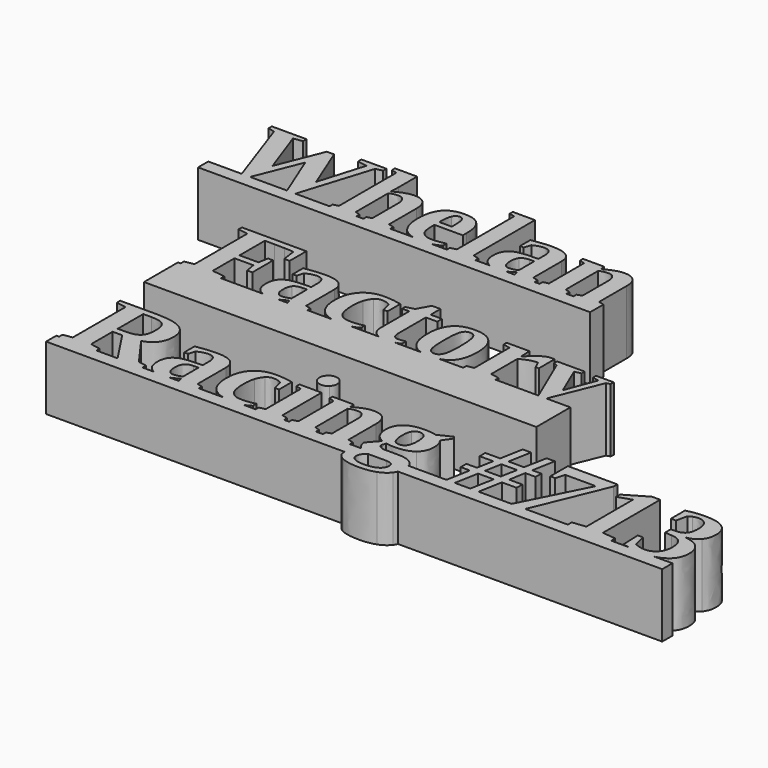
from build123d import *

# Parameters (mm, degrees)
F1_DEPTH = 15


with BuildPart() as f1:
    # F0 (on Top) → F1 (new body)
    with BuildSketch(Plane.XY):
        with BuildLine():
            Line((-29.6238354695, 35.7050479947), (-29.6238354695, 34.8109507725))
            Line((-29.6238354695, 34.8109507725), (-23.2913701918, 34.8109507725))
            Line((-23.2913701918, 34.8109507725), (-23.2913701918, 35.7050479947))
            Line((-23.2913701918, 35.7050479947), (-24.4545646362, 36.030568828))
            Line((-24.4545646362, 36.030568828), (-24.4545646362, 45.5661591058))
            add(Edge.make_bspline(
                [(-22.3929326918, 46.0262285502), (-23.4259188029, 46.0262285502), (-24.4545646362, 45.5661591058)],
                knots=[0, 0, 0, 1, 1, 1], degree=2))
            add(Edge.make_bspline(
                [(-21.0170646362, 45.3903778558), (-21.4988354695, 46.0262285502), (-22.3929326918, 46.0262285502)],
                knots=[0, 0, 0, 1, 1, 1], degree=2))
            add(Edge.make_bspline(
                [(-20.5352938029, 43.6130341058), (-20.5352938029, 44.7545271614), (-21.0170646362, 45.3903778558)],
                knots=[0, 0, 0, 1, 1, 1], degree=2))
            Line((-20.5352938029, 43.6130341058), (-20.5352938029, 36.030568828))
            Line((-20.5352938029, 36.030568828), (-21.6767868584, 35.7050479947))
            Line((-21.6767868584, 35.7050479947), (-21.6767868584, 34.8109507725))
            Line((-21.6767868584, 34.8109507725), (-15.3399813029, 34.8109507725))
            Line((-15.3399813029, 34.8109507725), (-15.3399813029, 35.7050479947))
            Line((-15.3399813029, 35.7050479947), (-16.6160229695, 36.030568828))
            Line((-16.6160229695, 36.030568828), (-16.6160229695, 44.1425479947))
            add(Edge.make_bspline(
                [(-20.1446688029, 47.9012285502), (-16.6160229695, 47.9012285502), (-16.6160229695, 44.1425479947)],
                knots=[0, 0, 0, 1, 1, 1], degree=2))
            add(Edge.make_bspline(
                [(-23.6038701918, 46.9246660502), (-21.6767868584, 47.9012285502), (-20.1446688029, 47.9012285502)],
                knots=[0, 0, 0, 1, 1, 1], degree=2))
            Line((-23.6038701918, 46.9246660502), (-24.537029914, 46.4472354947))
            add(Edge.make_bspline(
                [(-24.4545646362, 48.5652910502), (-24.4545646362, 47.671193828), (-24.537029914, 46.4472354947)],
                knots=[0, 0, 0, 1, 1, 1], degree=2))
            Line((-24.4545646362, 48.5652910502), (-24.4545646362, 54.0861243836))
            Line((-24.4545646362, 54.0861243836), (-29.6802590806, 54.0861243836))
            Line((-29.6802590806, 54.0861243836), (-29.6802590806, 53.1876868836))
            Line((-29.6802590806, 53.1876868836), (-28.3781757473, 52.8621660502))
            Line((-28.3781757473, 52.8621660502), (-28.3781757473, 36.030568828))
            Line((-28.3781757473, 36.030568828), (-29.6238354695, 35.7050479947))
        make_face()
        with BuildLine():
            Line((-23.2913701918, 34.8109507725), (-29.6238354695, 34.8109507725))
            Line((-29.6238354695, 34.8109507725), (-37.6563465286, 34.8109507725))
            Line((-37.6563465286, 34.8109507725), (-37.7878979695, 34.389943828))
            Line((-37.7878979695, 34.389943828), (-39.458904914, 34.389943828))
            Line((-39.458904914, 34.389943828), (-39.62877348, 34.8109507725))
            Line((-39.62877348, 34.8109507725), (-48.3094364931, 34.8109507725))
            Line((-48.3094364931, 34.8109507725), (-48.4780021362, 34.389943828))
            Line((-48.4780021362, 34.389943828), (-50.1446688029, 34.389943828))
            Line((-50.1446688029, 34.389943828), (-50.291566148, 34.8109507725))
            Line((-50.291566148, 34.8109507725), (-58.1481410251, 34.8109507725))
            Line((-58.1481410251, 34.8109507725), (-58.1481410251, 31.8109507725))
            Line((-58.1481410251, 31.8109507725), (34.0436992527, 31.8109507725))
            Line((34.0436992527, 31.8109507725), (34.0436992527, 34.8109507725))
            Line((34.0436992527, 34.8109507725), (27.7068936971, 34.8109507725))
            Line((27.7068936971, 34.8109507725), (26.0923103638, 34.8109507725))
            Line((26.0923103638, 34.8109507725), (19.759845086, 34.8109507725))
            Line((19.759845086, 34.8109507725), (18.5923103638, 34.8109507725))
            Line((18.5923103638, 34.8109507725), (13.900470086, 34.8109507725))
            Line((13.900470086, 34.8109507725), (11.7167314517, 34.8109507725))
            add(Edge.make_bspline(
                [(11.7167314517, 34.8109507725), (11.7028880575, 34.8065509266), (11.6890985582, 34.8022702169)],
                knots=[0.983831549, 0.983831549, 0.983831549, 1, 1, 1], degree=2))
            add(Edge.make_bspline(
                [(11.6890985582, 34.8022702169), (10.8362339749, 34.5375132725), (9.9681784194, 34.5375132725)],
                knots=[0, 0, 0, 1, 1, 1], degree=2))
            add(Edge.make_bspline(
                [(9.9681784194, 34.5375132725), (8.9089804507, 34.5375132725), (8.133832853, 34.8109507725)],
                knots=[0, 0, 0, 0.2681749582, 0.2681749582, 0.2681749582], degree=2))
            Line((8.133832853, 34.8109507725), (4.6513381416, 34.8109507725))
            Line((4.6513381416, 34.8109507725), (-2.0500507473, 34.8109507725))
            Line((-2.0500507473, 34.8109507725), (-5.6748044805, 34.8109507725))
            add(Edge.make_bspline(
                [(-5.6748044805, 34.8109507725), (-6.7853617712, 34.5548743836), (-7.8443215806, 34.5548743836)],
                knots=[0.061598692, 0.061598692, 0.061598692, 1, 1, 1], degree=2))
            add(Edge.make_bspline(
                [(-7.8443215806, 34.5548743836), (-9.0848257788, 34.5548743836), (-10.0689135132, 34.8109507725)],
                knots=[0, 0, 0, 0.3958617275, 0.3958617275, 0.3958617275], degree=2))
            Line((-10.0689135132, 34.8109507725), (-15.3399813029, 34.8109507725))
            Line((-15.3399813029, 34.8109507725), (-21.6767868584, 34.8109507725))
            Line((-21.6767868584, 34.8109507725), (-23.2913701918, 34.8109507725))
        make_face()
        Polygon((-37.7878979695, 34.389943828), (-37.6563465286, 34.8109507725), (-39.62877348, 34.8109507725), (-39.458904914, 34.389943828), align=None)
        Polygon((-39.62877348, 34.8109507725), (-37.6563465286, 34.8109507725), (-32.3929326918, 51.655568828), (-30.8043910251, 52.0114716058), (-30.8043910251, 53.0010549391), (-36.6898076918, 53.0010549391), (-36.6898076918, 52.0114716058), (-34.3981410251, 51.655568828), (-37.6142868584, 40.8482771614), (-41.8851201918, 51.4515757725), (-43.5821688029, 51.4515757725), (-47.8399813029, 40.8178952169), (-51.7201896362, 51.655568828), (-49.5891132473, 52.0114716058), (-49.5891132473, 53.0010549391), (-57.7531757473, 53.0010549391), (-57.7531757473, 52.0114716058), (-56.1689743584, 51.655568828), (-50.291566148, 34.8109507725), (-48.3094364931, 34.8109507725), (-43.9858146362, 45.6095618836), align=None)
        Polygon((-48.4780021362, 34.389943828), (-48.3094364931, 34.8109507725), (-50.291566148, 34.8109507725), (-50.1446688029, 34.389943828), align=None)
        with BuildLine():
            add(Edge.make_bspline(
                [(-10.0689135132, 34.8109507725), (-11.5707638375, 35.2017578055), (-12.4753979695, 36.1889889669)],
                knots=[0.3958617275, 0.3958617275, 0.3958617275, 1, 1, 1], degree=2))
            Line((-10.0689135132, 34.8109507725), (-5.6748044805, 34.8109507725))
            add(Edge.make_bspline(
                [(-5.5287833862, 34.8456729947), (-5.6019050974, 34.8277601806), (-5.6748044805, 34.8109507725)],
                knots=[0, 0, 0, 0.061598692, 0.061598692, 0.061598692], degree=2))
            add(Edge.make_bspline(
                [(-3.599529914, 35.5835202169), (-4.341717414, 35.1364716058), (-5.5287833862, 34.8456729947)],
                knots=[0, 0, 0, 1, 1, 1], degree=2))
            Line((-3.599529914, 35.5835202169), (-3.599529914, 36.6295271614))
            add(Edge.make_bspline(
                [(-6.607342414, 36.2345618836), (-5.4137660251, 36.2345618836), (-3.599529914, 36.6295271614)],
                knots=[0, 0, 0, 1, 1, 1], degree=2))
            add(Edge.make_bspline(
                [(-8.6168910251, 36.6816104947), (-7.8833840806, 36.2345618836), (-6.607342414, 36.2345618836)],
                knots=[0, 0, 0, 1, 1, 1], degree=2))
            add(Edge.make_bspline(
                [(-9.6759188029, 37.983693828), (-9.3503979695, 37.1286591058), (-8.6168910251, 36.6816104947)],
                knots=[0, 0, 0, 1, 1, 1], degree=2))
            add(Edge.make_bspline(
                [(-10.0014396362, 40.8612979947), (-10.0014396362, 38.8387285502), (-9.6759188029, 37.983693828)],
                knots=[0, 0, 0, 1, 1, 1], degree=2))
            Line((-10.0014396362, 40.8612979947), (-10.0014396362, 41.0783118836))
            Line((-10.0014396362, 41.0783118836), (-3.3130715806, 41.0783118836))
            Line((-3.3130715806, 41.0783118836), (-3.3130715806, 42.1894229947))
            add(Edge.make_bspline(
                [(-4.4719257473, 46.4884681336), (-3.3130715806, 45.1060896614), (-3.3130715806, 42.1894229947)],
                knots=[0, 0, 0, 1, 1, 1], degree=2))
            add(Edge.make_bspline(
                [(-8.2219257473, 47.8708466058), (-5.630779914, 47.8708466058), (-4.4719257473, 46.4884681336)],
                knots=[0, 0, 0, 1, 1, 1], degree=2))
            add(Edge.make_bspline(
                [(-12.5426722751, 46.2302216058), (-11.1125507473, 47.8708466058), (-8.2219257473, 47.8708466058)],
                knots=[0, 0, 0, 1, 1, 1], degree=2))
            add(Edge.make_bspline(
                [(-13.9727938029, 41.2519229947), (-13.9727938029, 44.5895966058), (-12.5426722751, 46.2302216058)],
                knots=[0, 0, 0, 1, 1, 1], degree=2))
            add(Edge.make_bspline(
                [(-12.4753979695, 36.1889889669), (-13.9727938029, 37.8231035502), (-13.9727938029, 41.2519229947)],
                knots=[0, 0, 0, 1, 1, 1], degree=2))
        make_face()
        with BuildLine():
            add(Edge.make_bspline(
                [(-8.3738354695, 46.5036591058), (-9.185467414, 46.5036591058), (-9.5847729695, 45.6225827169)],
                knots=[0, 0, 0, 1, 1, 1], degree=2))
            add(Edge.make_bspline(
                [(-7.564373664, 46.1499264669), (-7.857342414, 46.5036591058), (-8.3738354695, 46.5036591058)],
                knots=[0, 0, 0, 1, 1, 1], degree=2))
            add(Edge.make_bspline(
                [(-7.1498771362, 45.0583466058), (-7.271404914, 45.796193828), (-7.564373664, 46.1499264669)],
                knots=[0, 0, 0, 1, 1, 1], degree=2))
            add(Edge.make_bspline(
                [(-7.0283493584, 42.5019229947), (-7.0283493584, 44.3204993836), (-7.1498771362, 45.0583466058)],
                knots=[0, 0, 0, 1, 1, 1], degree=2))
            Line((-7.0283493584, 42.5019229947), (-9.9840785251, 42.5019229947))
            add(Edge.make_bspline(
                [(-9.5847729695, 45.6225827169), (-9.9840785251, 44.741506328), (-9.9840785251, 42.5019229947)],
                knots=[0, 0, 0, 1, 1, 1], degree=2))
        make_face(mode=Mode.SUBTRACT)
        with BuildLine():
            Line((-5.6748044805, 34.8109507725), (-10.0689135132, 34.8109507725))
            add(Edge.make_bspline(
                [(-7.8443215806, 34.5548743836), (-9.0848257788, 34.5548743836), (-10.0689135132, 34.8109507725)],
                knots=[0, 0, 0, 0.3958617275, 0.3958617275, 0.3958617275], degree=2))
            add(Edge.make_bspline(
                [(-5.6748044805, 34.8109507725), (-6.7853617712, 34.5548743836), (-7.8443215806, 34.5548743836)],
                knots=[0.061598692, 0.061598692, 0.061598692, 1, 1, 1], degree=2))
        make_face()
        Polygon((-2.0500507473, 35.7050479947), (-2.0500507473, 34.8109507725), (4.6513381416, 34.8109507725), (4.6513381416, 35.7050479947), (3.2537686971, 36.030568828), (3.2537686971, 54.0861243836), (-1.9675854695, 54.0861243836), (-1.9675854695, 53.1876868836), (-0.6655021362, 52.8621660502), (-0.6655021362, 36.030568828), align=None)
        with BuildLine():
            add(Edge.make_bspline(
                [(8.133832853, 34.8109507725), (6.0185256416, 35.5571368116), (6.0185256416, 38.3395966058)],
                knots=[0.2681749582, 0.2681749582, 0.2681749582, 1, 1, 1], degree=2))
            Line((8.133832853, 34.8109507725), (11.7167314517, 34.8109507725))
            add(Edge.make_bspline(
                [(13.6009909194, 35.7875132725), (12.5590859803, 35.0786763058), (11.7167314517, 34.8109507725)],
                knots=[0, 0, 0, 0.983831549, 0.983831549, 0.983831549], degree=2))
            Line((13.6009909194, 35.7875132725), (13.900470086, 34.8109507725))
            Line((13.900470086, 34.8109507725), (18.5923103638, 34.8109507725))
            Line((18.5923103638, 34.8109507725), (18.5923103638, 35.7050479947))
            Line((18.5923103638, 35.7050479947), (17.3162686971, 36.030568828))
            Line((17.3162686971, 36.030568828), (17.3162686971, 44.3204993836))
            add(Edge.make_bspline(
                [(12.5289423082, 47.8448049391), (17.3162686971, 47.8448049391), (17.3162686971, 44.3204993836)],
                knots=[0, 0, 0, 1, 1, 1], degree=2))
            add(Edge.make_bspline(
                [(10.5627964749, 47.7645098002), (11.5263381416, 47.8448049391), (12.5289423082, 47.8448049391)],
                knots=[0, 0, 0, 1, 1, 1], degree=2))
            add(Edge.make_bspline(
                [(7.5506436971, 47.3717146614), (9.5992548082, 47.6842146614), (10.5627964749, 47.7645098002)],
                knots=[0, 0, 0, 1, 1, 1], degree=2))
            Line((7.5506436971, 47.3717146614), (7.5506436971, 44.2901174391))
            Line((7.5506436971, 44.2901174391), (8.4490811971, 44.2901174391))
            Line((8.4490811971, 44.2901174391), (8.9612339749, 45.8786591058))
            add(Edge.make_bspline(
                [(11.5133173082, 46.5861243836), (10.3718242527, 46.5861243836), (8.9612339749, 45.8786591058)],
                knots=[0, 0, 0, 1, 1, 1], degree=2))
            add(Edge.make_bspline(
                [(13.3969978638, 44.2770966058), (13.3969978638, 46.5861243836), (11.5133173082, 46.5861243836)],
                knots=[0, 0, 0, 1, 1, 1], degree=2))
            Line((13.3969978638, 44.2770966058), (13.3969978638, 42.4194577169))
            Line((13.3969978638, 42.4194577169), (11.7433520305, 42.3803952169))
            add(Edge.make_bspline(
                [(8.2841506416, 41.9116452169), (9.3822409194, 42.3239716058), (11.7433520305, 42.3803952169)],
                knots=[0, 0, 0, 1, 1, 1], degree=2))
            add(Edge.make_bspline(
                [(6.6022930027, 40.6377736891), (7.1860603638, 41.499318828), (8.2841506416, 41.9116452169)],
                knots=[0, 0, 0, 1, 1, 1], degree=2))
            add(Edge.make_bspline(
                [(6.0185256416, 38.3395966058), (6.0185256416, 39.7762285502), (6.6022930027, 40.6377736891)],
                knots=[0, 0, 0, 1, 1, 1], degree=2))
        make_face()
        with BuildLine():
            Line((12.259845086, 41.1737979947), (13.3969978638, 41.2128604947))
            Line((13.3969978638, 41.2128604947), (13.3969978638, 36.655568828))
            add(Edge.make_bspline(
                [(11.3917895305, 36.1824785502), (12.3119284194, 36.1824785502), (13.3969978638, 36.655568828)],
                knots=[0, 0, 0, 1, 1, 1], degree=2))
            add(Edge.make_bspline(
                [(10.3327617527, 36.7250132725), (10.7407478638, 36.1824785502), (11.3917895305, 36.1824785502)],
                knots=[0, 0, 0, 1, 1, 1], degree=2))
            add(Edge.make_bspline(
                [(9.9247756416, 38.4177216058), (9.9247756416, 37.2675479947), (10.3327617527, 36.7250132725)],
                knots=[0, 0, 0, 1, 1, 1], degree=2))
            add(Edge.make_bspline(
                [(10.4347582805, 40.4793535502), (9.9247756416, 39.8413327169), (9.9247756416, 38.4177216058)],
                knots=[0, 0, 0, 1, 1, 1], degree=2))
            add(Edge.make_bspline(
                [(12.259845086, 41.1737979947), (10.9447409194, 41.1173743836), (10.4347582805, 40.4793535502)],
                knots=[0, 0, 0, 1, 1, 1], degree=2))
        make_face(mode=Mode.SUBTRACT)
        with BuildLine():
            Line((11.7167314517, 34.8109507725), (8.133832853, 34.8109507725))
            add(Edge.make_bspline(
                [(9.9681784194, 34.5375132725), (8.9089804507, 34.5375132725), (8.133832853, 34.8109507725)],
                knots=[0, 0, 0, 0.2681749582, 0.2681749582, 0.2681749582], degree=2))
            add(Edge.make_bspline(
                [(11.6890985582, 34.8022702169), (10.8362339749, 34.5375132725), (9.9681784194, 34.5375132725)],
                knots=[0, 0, 0, 1, 1, 1], degree=2))
            add(Edge.make_bspline(
                [(11.7167314517, 34.8109507725), (11.7028880575, 34.8065509266), (11.6890985582, 34.8022702169)],
                knots=[0.983831549, 0.983831549, 0.983831549, 1, 1, 1], degree=2))
        make_face()
        with BuildLine():
            Line((27.7068936971, 34.8109507725), (34.0436992527, 34.8109507725))
            Line((34.0436992527, 34.8109507725), (34.0436992527, 35.7050479947))
            Line((34.0436992527, 35.7050479947), (32.767657586, 36.030568828))
            Line((32.767657586, 36.030568828), (32.767657586, 44.1425479947))
            add(Edge.make_bspline(
                [(29.2390117527, 47.9012285502), (32.767657586, 47.9012285502), (32.767657586, 44.1425479947)],
                knots=[0, 0, 0, 1, 1, 1], degree=2))
            add(Edge.make_bspline(
                [(25.8232131416, 46.9246660502), (27.7199145305, 47.9012285502), (29.2390117527, 47.9012285502)],
                knots=[0, 0, 0, 1, 1, 1], degree=2))
            Line((25.8232131416, 46.9246660502), (24.8987339749, 46.4472354947))
            Line((24.8987339749, 46.4472354947), (24.7121020305, 47.5626868836))
            Line((24.7121020305, 47.5626868836), (19.759845086, 47.5626868836))
            Line((19.759845086, 47.5626868836), (19.759845086, 46.6642493836))
            Line((19.759845086, 46.6642493836), (21.0055048082, 46.3387285502))
            Line((21.0055048082, 46.3387285502), (21.0055048082, 36.030568828))
            Line((21.0055048082, 36.030568828), (19.759845086, 35.7050479947))
            Line((19.759845086, 35.7050479947), (19.759845086, 34.8109507725))
            Line((19.759845086, 34.8109507725), (26.0923103638, 34.8109507725))
            Line((26.0923103638, 34.8109507725), (26.0923103638, 35.7050479947))
            Line((26.0923103638, 35.7050479947), (24.9291159194, 36.030568828))
            Line((24.9291159194, 36.030568828), (24.9291159194, 45.5661591058))
            add(Edge.make_bspline(
                [(26.9907478638, 46.0262285502), (25.9577617527, 46.0262285502), (24.9291159194, 45.5661591058)],
                knots=[0, 0, 0, 1, 1, 1], degree=2))
            add(Edge.make_bspline(
                [(28.3666159194, 45.3903778558), (27.884845086, 46.0262285502), (26.9907478638, 46.0262285502)],
                knots=[0, 0, 0, 1, 1, 1], degree=2))
            add(Edge.make_bspline(
                [(28.8483867527, 43.6130341058), (28.8483867527, 44.7545271614), (28.3666159194, 45.3903778558)],
                knots=[0, 0, 0, 1, 1, 1], degree=2))
            Line((28.8483867527, 43.6130341058), (28.8483867527, 36.030568828))
            Line((28.8483867527, 36.030568828), (27.7068936971, 35.7050479947))
            Line((27.7068936971, 35.7050479947), (27.7068936971, 34.8109507725))
        make_face()
        with BuildLine():
            Line((-36.774163597, 0), (-37.4252052637, 0))
            Line((-37.4252052637, 0), (-37.4252052637, -10))
            Line((-37.4252052637, -10), (54.8491002919, -10))
            Line((54.8491002919, -10), (54.8491002919, 0))
            Line((54.8491002919, 0), (49.2186661972, 0))
            Line((49.2186661972, 0), (48.8942391808, -0.7986111111))
            add(Edge.make_bspline(
                [(48.8942391808, -0.7986111111), (48.0261836252, -3.0121527778), (47.3751419586, -4.0082465278)],
                knots=[0, 0, 0, 1, 1, 1], degree=2))
            add(Edge.make_bspline(
                [(47.3751419586, -4.0082465278), (46.7241002919, -5.0043402778), (45.9298294586, -5.4991319444)],
                knots=[0, 0, 0, 1, 1, 1], degree=2))
            add(Edge.make_bspline(
                [(45.9298294586, -5.4991319444), (45.1355586252, -5.9939236111), (44.1199336252, -5.9939236111)],
                knots=[0, 0, 0, 1, 1, 1], degree=2))
            add(Edge.make_bspline(
                [(44.1199336252, -5.9939236111), (43.0218433474, -5.9939236111), (41.8803502919, -5.7378472222)],
                knots=[0, 0, 0, 1, 1, 1], degree=2))
            Line((41.8803502919, -5.7378472222), (41.8803502919, -2.4565972222))
            Line((41.8803502919, -2.4565972222), (42.6963225141, -2.4565972222))
            Line((42.6963225141, -2.4565972222), (43.2779197363, -4.1623263889))
            add(Edge.make_bspline(
                [(43.2779197363, -4.1623263889), (43.6728850141, -4.4748263889), (44.280523903, -4.4748263889)],
                knots=[0, 0, 0, 1, 1, 1], degree=2))
            add(Edge.make_bspline(
                [(44.280523903, -4.4748263889), (44.7970169586, -4.4748263889), (45.1898120974, -4.2317708333)],
                knots=[0, 0, 0, 1, 1, 1], degree=2))
            add(Edge.make_bspline(
                [(45.1898120974, -4.2317708333), (45.5826072363, -3.9887152778), (45.9298294586, -3.5264756944)],
                knots=[0, 0, 0, 1, 1, 1], degree=2))
            add(Edge.make_bspline(
                [(45.9298294586, -3.5264756944), (46.2770516808, -3.0642361111), (46.5873815419, -2.3936631944)],
                knots=[0, 0, 0, 1, 1, 1], degree=2))
            add(Edge.make_bspline(
                [(46.5873815419, -2.3936631944), (46.897711403, -1.7230902778), (47.4966697363, -0.3949652778)],
                knots=[0, 0, 0, 1, 1, 1], degree=2))
            Line((47.4966697363, -0.3949652778), (47.3277275443, 0))
            Line((47.3277275443, 0), (37.2666350141, 0))
            Line((37.2666350141, 0), (29.6451072363, 0))
            Line((29.6451072363, 0), (24.0814538313, 0))
            add(Edge.make_bspline(
                [(24.0814538313, 0), (23.1058756874, -0.2734375), (21.8716697363, -0.2734375)],
                knots=[0.5920214475, 0.5920214475, 0.5920214475, 1, 1, 1], degree=2))
            add(Edge.make_bspline(
                [(21.8716697363, -0.2734375), (20.6834625195, -0.2734375), (19.7408492975, 0)],
                knots=[0, 0, 0, 0.40557473, 0.40557473, 0.40557473], degree=2))
            Line((19.7408492975, 0), (13.6655846372, 0))
            add(Edge.make_bspline(
                [(13.6655846372, 0), (13.5835685904, -0.0208093797), (13.4971037641, -0.0412326389)],
                knots=[0.9120463753, 0.9120463753, 0.9120463753, 1, 1, 1], degree=2))
            add(Edge.make_bspline(
                [(13.4971037641, -0.0412326389), (12.5140308474, -0.2734375), (11.702398903, -0.2734375)],
                knots=[0, 0, 0, 1, 1, 1], degree=2))
            add(Edge.make_bspline(
                [(11.702398903, -0.2734375), (10.6504768322, -0.2734375), (9.8741396763, 0)],
                knots=[0, 0, 0, 0.5743195382, 0.5743195382, 0.5743195382], degree=2))
            Line((9.8741396763, 0), (3.318596057, 0))
            add(Edge.make_bspline(
                [(3.318596057, 0), (2.26893498, -0.2560763889), (1.1598641808, -0.2560763889)],
                knots=[0.0284033759, 0.0284033759, 0.0284033759, 1, 1, 1], degree=2))
            add(Edge.make_bspline(
                [(1.1598641808, -0.2560763889), (-0.1844899744, -0.2560763889), (-1.2612510776, 0)],
                knots=[0, 0, 0, 0.3950755068, 0.3950755068, 0.3950755068], degree=2))
            Line((-1.2612510776, 0), (-6.9911774859, 0))
            Line((-6.9911774859, 0), (-11.6830177637, 0))
            Line((-11.6830177637, 0), (-13.866756398, 0))
            add(Edge.make_bspline(
                [(-13.866756398, 0), (-13.8805997922, -0.0043998459), (-13.8943892914, -0.0086805556)],
                knots=[0.983831549, 0.983831549, 0.983831549, 1, 1, 1], degree=2))
            add(Edge.make_bspline(
                [(-13.8943892914, -0.0086805556), (-14.7472538748, -0.2734375), (-15.6153094303, -0.2734375)],
                knots=[0, 0, 0, 1, 1, 1], degree=2))
            add(Edge.make_bspline(
                [(-15.6153094303, -0.2734375), (-16.674507399, -0.2734375), (-17.4496549967, 0)],
                knots=[0, 0, 0, 0.2681749582, 0.2681749582, 0.2681749582], degree=2))
            Line((-17.4496549967, 0), (-27.321038597, 0))
            Line((-27.321038597, 0), (-36.774163597, 0))
        make_face()
        with BuildLine():
            Line((-36.774163597, 0.9895833333), (-36.774163597, 0))
            Line((-36.774163597, 0), (-27.321038597, 0))
            Line((-27.321038597, 0), (-27.321038597, 0.9895833333))
            Line((-27.321038597, 0.9895833333), (-30.3462122081, 1.3585069444))
            Line((-30.3462122081, 1.3585069444), (-30.3462122081, 7.7604166667))
            Line((-30.3462122081, 7.7604166667), (-25.9104483192, 7.7604166667))
            Line((-25.9104483192, 7.7604166667), (-25.4894413748, 5.4253472222))
            Line((-25.4894413748, 5.4253472222), (-24.2828441526, 5.4253472222))
            Line((-24.2828441526, 5.4253472222), (-24.2828441526, 11.5581597222))
            Line((-24.2828441526, 11.5581597222), (-25.4894413748, 11.5581597222))
            Line((-25.4894413748, 11.5581597222), (-25.9104483192, 9.2491319444))
            Line((-25.9104483192, 9.2491319444), (-30.3462122081, 9.2491319444))
            Line((-30.3462122081, 9.2491319444), (-30.3462122081, 16.6970486111))
            Line((-30.3462122081, 16.6970486111), (-28.1066288748, 16.6970486111))
            add(Edge.make_bspline(
                [(-25.6934344303, 16.6493055556), (-27.2255524859, 16.6970486111), (-28.1066288748, 16.6970486111)],
                knots=[0, 0, 0, 1, 1, 1], degree=2))
            add(Edge.make_bspline(
                [(-23.4972538748, 16.5060763889), (-24.1613163748, 16.6015625), (-25.6934344303, 16.6493055556)],
                knots=[0, 0, 0, 1, 1, 1], degree=2))
            Line((-23.4972538748, 16.5060763889), (-23.063226097, 13.2942708333))
            Line((-23.063226097, 13.2942708333), (-21.7871844303, 13.2942708333))
            Line((-21.7871844303, 13.2942708333), (-21.7871844303, 18.1901041667))
            Line((-21.7871844303, 18.1901041667), (-36.9521149859, 18.1901041667))
            Line((-36.9521149859, 18.1901041667), (-36.9521149859, 17.2005208333))
            Line((-36.9521149859, 17.2005208333), (-34.6170455414, 16.8446180556))
            Line((-34.6170455414, 16.8446180556), (-34.6170455414, 1.3585069444))
            Line((-34.6170455414, 1.3585069444), (-36.774163597, 0.9895833333))
        make_face()
        with BuildLine():
            add(Edge.make_bspline(
                [(-17.4496549967, 0), (-19.5649622081, 0.7461860391), (-19.5649622081, 3.5286458333)],
                knots=[0.2681749582, 0.2681749582, 0.2681749582, 1, 1, 1], degree=2))
            Line((-17.4496549967, 0), (-13.866756398, 0))
            add(Edge.make_bspline(
                [(-11.9824969303, 0.9765625), (-13.0244018694, 0.2677255333), (-13.866756398, 0)],
                knots=[0, 0, 0, 0.983831549, 0.983831549, 0.983831549], degree=2))
            Line((-11.9824969303, 0.9765625), (-11.6830177637, 0))
            Line((-11.6830177637, 0), (-6.9911774859, 0))
            Line((-6.9911774859, 0), (-6.9911774859, 0.8940972222))
            Line((-6.9911774859, 0.8940972222), (-8.2672191526, 1.2196180556))
            Line((-8.2672191526, 1.2196180556), (-8.2672191526, 9.5095486111))
            add(Edge.make_bspline(
                [(-13.0545455414, 13.0338541667), (-8.2672191526, 13.0338541667), (-8.2672191526, 9.5095486111)],
                knots=[0, 0, 0, 1, 1, 1], degree=2))
            add(Edge.make_bspline(
                [(-15.0206913748, 12.9535590278), (-14.0571497081, 13.0338541667), (-13.0545455414, 13.0338541667)],
                knots=[0, 0, 0, 1, 1, 1], degree=2))
            add(Edge.make_bspline(
                [(-18.0328441526, 12.5607638889), (-15.9842330414, 12.8732638889), (-15.0206913748, 12.9535590278)],
                knots=[0, 0, 0, 1, 1, 1], degree=2))
            Line((-18.0328441526, 12.5607638889), (-18.0328441526, 9.4791666667))
            Line((-18.0328441526, 9.4791666667), (-17.1344066526, 9.4791666667))
            Line((-17.1344066526, 9.4791666667), (-16.6222538748, 11.0677083333))
            add(Edge.make_bspline(
                [(-14.0701705414, 11.7751736111), (-15.211663597, 11.7751736111), (-16.6222538748, 11.0677083333)],
                knots=[0, 0, 0, 1, 1, 1], degree=2))
            add(Edge.make_bspline(
                [(-12.1864899859, 9.4661458333), (-12.1864899859, 11.7751736111), (-14.0701705414, 11.7751736111)],
                knots=[0, 0, 0, 1, 1, 1], degree=2))
            Line((-12.1864899859, 9.4661458333), (-12.1864899859, 7.6085069444))
            Line((-12.1864899859, 7.6085069444), (-13.8401358192, 7.5694444444))
            add(Edge.make_bspline(
                [(-17.2993372081, 7.1006944444), (-16.2012469303, 7.5130208333), (-13.8401358192, 7.5694444444)],
                knots=[0, 0, 0, 1, 1, 1], degree=2))
            add(Edge.make_bspline(
                [(-18.981194847, 5.8268229167), (-18.3974274859, 6.6883680556), (-17.2993372081, 7.1006944444)],
                knots=[0, 0, 0, 1, 1, 1], degree=2))
            add(Edge.make_bspline(
                [(-19.5649622081, 3.5286458333), (-19.5649622081, 4.9652777778), (-18.981194847, 5.8268229167)],
                knots=[0, 0, 0, 1, 1, 1], degree=2))
        make_face()
        with BuildLine():
            Line((-13.3236427637, 6.3628472222), (-12.1864899859, 6.4019097222))
            Line((-12.1864899859, 6.4019097222), (-12.1864899859, 1.8446180556))
            add(Edge.make_bspline(
                [(-14.1916983192, 1.3715277778), (-13.2715594303, 1.3715277778), (-12.1864899859, 1.8446180556)],
                knots=[0, 0, 0, 1, 1, 1], degree=2))
            add(Edge.make_bspline(
                [(-15.250726097, 1.9140625), (-14.8427399859, 1.3715277778), (-14.1916983192, 1.3715277778)],
                knots=[0, 0, 0, 1, 1, 1], degree=2))
            add(Edge.make_bspline(
                [(-15.6587122081, 3.6067708333), (-15.6587122081, 2.4565972222), (-15.250726097, 1.9140625)],
                knots=[0, 0, 0, 1, 1, 1], degree=2))
            add(Edge.make_bspline(
                [(-15.1487295692, 5.6684027778), (-15.6587122081, 5.0303819444), (-15.6587122081, 3.6067708333)],
                knots=[0, 0, 0, 1, 1, 1], degree=2))
            add(Edge.make_bspline(
                [(-13.3236427637, 6.3628472222), (-14.6387469303, 6.3064236111), (-15.1487295692, 5.6684027778)],
                knots=[0, 0, 0, 1, 1, 1], degree=2))
        make_face(mode=Mode.SUBTRACT)
        with BuildLine():
            Line((-13.866756398, 0), (-17.4496549967, 0))
            add(Edge.make_bspline(
                [(-15.6153094303, -0.2734375), (-16.674507399, -0.2734375), (-17.4496549967, 0)],
                knots=[0, 0, 0, 0.2681749582, 0.2681749582, 0.2681749582], degree=2))
            add(Edge.make_bspline(
                [(-13.8943892914, -0.0086805556), (-14.7472538748, -0.2734375), (-15.6153094303, -0.2734375)],
                knots=[0, 0, 0, 1, 1, 1], degree=2))
            add(Edge.make_bspline(
                [(-13.866756398, 0), (-13.8805997922, -0.0043998459), (-13.8943892914, -0.0086805556)],
                knots=[0.983831549, 0.983831549, 0.983831549, 1, 1, 1], degree=2))
        make_face()
        with BuildLine():
            Line((48.8942391808, -0.7986111111), (49.2186661972, 0))
            Line((49.2186661972, 0), (47.3277275443, 0))
            Line((47.3277275443, 0), (47.4966697363, -0.3949652778))
            add(Edge.make_bspline(
                [(46.5873815419, -2.3936631944), (46.897711403, -1.7230902778), (47.4966697363, -0.3949652778)],
                knots=[0, 0, 0, 1, 1, 1], degree=2))
            add(Edge.make_bspline(
                [(45.9298294586, -3.5264756944), (46.2770516808, -3.0642361111), (46.5873815419, -2.3936631944)],
                knots=[0, 0, 0, 1, 1, 1], degree=2))
            add(Edge.make_bspline(
                [(45.1898120974, -4.2317708333), (45.5826072363, -3.9887152778), (45.9298294586, -3.5264756944)],
                knots=[0, 0, 0, 1, 1, 1], degree=2))
            add(Edge.make_bspline(
                [(44.280523903, -4.4748263889), (44.7970169586, -4.4748263889), (45.1898120974, -4.2317708333)],
                knots=[0, 0, 0, 1, 1, 1], degree=2))
            add(Edge.make_bspline(
                [(43.2779197363, -4.1623263889), (43.6728850141, -4.4748263889), (44.280523903, -4.4748263889)],
                knots=[0, 0, 0, 1, 1, 1], degree=2))
            Line((43.2779197363, -4.1623263889), (42.6963225141, -2.4565972222))
            Line((42.6963225141, -2.4565972222), (41.8803502919, -2.4565972222))
            Line((41.8803502919, -2.4565972222), (41.8803502919, -5.7378472222))
            add(Edge.make_bspline(
                [(44.1199336252, -5.9939236111), (43.0218433474, -5.9939236111), (41.8803502919, -5.7378472222)],
                knots=[0, 0, 0, 1, 1, 1], degree=2))
            add(Edge.make_bspline(
                [(45.9298294586, -5.4991319444), (45.1355586252, -5.9939236111), (44.1199336252, -5.9939236111)],
                knots=[0, 0, 0, 1, 1, 1], degree=2))
            add(Edge.make_bspline(
                [(47.3751419586, -4.0082465278), (46.7241002919, -5.0043402778), (45.9298294586, -5.4991319444)],
                knots=[0, 0, 0, 1, 1, 1], degree=2))
            add(Edge.make_bspline(
                [(48.8942391808, -0.7986111111), (48.0261836252, -3.0121527778), (47.3751419586, -4.0082465278)],
                knots=[0, 0, 0, 1, 1, 1], degree=2))
        make_face()
        Polygon((47.3277275443, 0), (49.2186661972, 0), (53.9246211252, 11.5842013889), (54.8491002919, 11.8532986111), (54.8491002919, 12.7517361111), (50.6824336252, 12.7517361111), (50.6824336252, 11.8532986111), (52.1754891808, 11.5277777778), (49.5018780697, 4.4487847222), (46.507086403, 11.5017361111), (48.0261836252, 11.8532986111), (48.0261836252, 12.7517361111), (41.5027461252, 12.7517361111), (41.5027461252, 11.8532986111), (42.3968433474, 11.5277777778), align=None)
        with BuildLine():
            Line((29.6451072363, 0), (37.2666350141, 0))
            Line((37.2666350141, 0), (37.2666350141, 0.8940972222))
            Line((37.2666350141, 0.8940972222), (35.218023903, 1.2196180556))
            Line((35.218023903, 1.2196180556), (35.218023903, 8.9670138889))
            add(Edge.make_bspline(
                [(37.132086403, 9.8394097222), (36.0470169586, 9.4661458333), (35.218023903, 8.9670138889)],
                knots=[0, 0, 0, 1, 1, 1], degree=2))
            add(Edge.make_bspline(
                [(39.0721905697, 10.2126736111), (38.2171558474, 10.2126736111), (37.132086403, 9.8394097222)],
                knots=[0, 0, 0, 1, 1, 1], degree=2))
            Line((39.0721905697, 10.2126736111), (39.8708016808, 8.5026041667))
            Line((39.8708016808, 8.5026041667), (40.6303502919, 8.5026041667))
            Line((40.6303502919, 8.5026041667), (40.6303502919, 13.1553819444))
            Line((40.6303502919, 13.1553819444), (39.8968433474, 13.1553819444))
            add(Edge.make_bspline(
                [(37.776617653, 12.4435763889), (38.9376419586, 13.1553819444), (39.8968433474, 13.1553819444)],
                knots=[0, 0, 0, 1, 1, 1], degree=2))
            add(Edge.make_bspline(
                [(35.1529197363, 10.1041666667), (36.6155933474, 11.7317708333), (37.776617653, 12.4435763889)],
                knots=[0, 0, 0, 1, 1, 1], degree=2))
            Line((35.1529197363, 10.1041666667), (35.0010100141, 12.7517361111))
            Line((35.0010100141, 12.7517361111), (29.6451072363, 12.7517361111))
            Line((29.6451072363, 12.7517361111), (29.6451072363, 11.8532986111))
            Line((29.6451072363, 11.8532986111), (31.2987530697, 11.5277777778))
            Line((31.2987530697, 11.5277777778), (31.2987530697, 1.2196180556))
            Line((31.2987530697, 1.2196180556), (29.6451072363, 0.8940972222))
            Line((29.6451072363, 0.8940972222), (29.6451072363, 0))
        make_face()
        with BuildLine():
            add(Edge.make_bspline(
                [(-1.2612510776, 0), (-2.9099464622, 0.3920943645), (-3.9312816526, 1.3845486111)],
                knots=[0.3950755068, 0.3950755068, 0.3950755068, 1, 1, 1], degree=2))
            Line((-1.2612510776, 0), (3.318596057, 0))
            add(Edge.make_bspline(
                [(3.3799162641, 0.0151909722), (3.3492815466, 0.0074860634), (3.318596057, 0)],
                knots=[0, 0, 0, 0.0284033759, 0.0284033759, 0.0284033759], degree=2))
            add(Edge.make_bspline(
                [(5.0661141808, 0.7725694444), (4.4584752919, 0.2864583333), (3.3799162641, 0.0151909722)],
                knots=[0, 0, 0, 1, 1, 1], degree=2))
            Line((5.0661141808, 0.7725694444), (5.0661141808, 1.8185763889))
            add(Edge.make_bspline(
                [(1.8673294586, 1.4236111111), (3.7379891808, 1.4236111111), (5.0661141808, 1.8185763889)],
                knots=[0, 0, 0, 1, 1, 1], degree=2))
            add(Edge.make_bspline(
                [(-0.8258129026, 2.5911458333), (0.022711403, 1.4236111111), (1.8673294586, 1.4236111111)],
                knots=[0, 0, 0, 1, 1, 1], degree=2))
            add(Edge.make_bspline(
                [(-1.6743372081, 6.484375), (-1.6743372081, 3.7586805556), (-0.8258129026, 2.5911458333)],
                knots=[0, 0, 0, 1, 1, 1], degree=2))
            add(Edge.make_bspline(
                [(-1.3140941526, 9.2578125), (-1.6743372081, 8.0989583333), (-1.6743372081, 6.484375)],
                knots=[0, 0, 0, 1, 1, 1], degree=2))
            add(Edge.make_bspline(
                [(-0.3028094303, 11.0546875), (-0.953851097, 10.4166666667), (-1.3140941526, 9.2578125)],
                knots=[0, 0, 0, 1, 1, 1], degree=2))
            add(Edge.make_bspline(
                [(1.1468433474, 11.6927083333), (0.3482322363, 11.6927083333), (-0.3028094303, 11.0546875)],
                knots=[0, 0, 0, 1, 1, 1], degree=2))
            add(Edge.make_bspline(
                [(2.327398903, 11.5559895833), (1.8803502919, 11.6927083333), (1.1468433474, 11.6927083333)],
                knots=[0, 0, 0, 1, 1, 1], degree=2))
            add(Edge.make_bspline(
                [(3.2345169586, 11.0807291667), (2.7744475141, 11.4192708333), (2.327398903, 11.5559895833)],
                knots=[0, 0, 0, 1, 1, 1], degree=2))
            Line((3.2345169586, 11.0807291667), (3.8074336252, 8.8454861111))
            Line((3.8074336252, 8.8454861111), (4.7839961252, 8.8454861111))
            Line((4.7839961252, 8.8454861111), (4.7839961252, 12.6128472222))
            add(Edge.make_bspline(
                [(0.647711403, 13.0902777778), (2.5444127919, 13.0902777778), (4.7839961252, 12.6128472222)],
                knots=[0, 0, 0, 1, 1, 1], degree=2))
            add(Edge.make_bspline(
                [(-2.6639205414, 12.2960069444), (-1.2403094303, 13.0902777778), (0.647711403, 13.0902777778)],
                knots=[0, 0, 0, 1, 1, 1], degree=2))
            add(Edge.make_bspline(
                [(-4.8535906803, 10.0021701389), (-4.0875316526, 11.5017361111), (-2.6639205414, 12.2960069444)],
                knots=[0, 0, 0, 1, 1, 1], degree=2))
            add(Edge.make_bspline(
                [(-5.6196497081, 6.4019097222), (-5.6196497081, 8.5026041667), (-4.8535906803, 10.0021701389)],
                knots=[0, 0, 0, 1, 1, 1], degree=2))
            add(Edge.make_bspline(
                [(-3.9312816526, 1.3845486111), (-5.6196497081, 3.0251736111), (-5.6196497081, 6.4019097222)],
                knots=[0, 0, 0, 1, 1, 1], degree=2))
        make_face()
        with BuildLine():
            Line((3.318596057, 0), (-1.2612510776, 0))
            add(Edge.make_bspline(
                [(1.1598641808, -0.2560763889), (-0.1844899744, -0.2560763889), (-1.2612510776, 0)],
                knots=[0, 0, 0, 0.3950755068, 0.3950755068, 0.3950755068], degree=2))
            add(Edge.make_bspline(
                [(3.318596057, 0), (2.26893498, -0.2560763889), (1.1598641808, -0.2560763889)],
                knots=[0.0284033759, 0.0284033759, 0.0284033759, 1, 1, 1], degree=2))
        make_face()
        with BuildLine():
            add(Edge.make_bspline(
                [(24.0814538313, 0), (23.1058756874, -0.2734375), (21.8716697363, -0.2734375)],
                knots=[0.5920214475, 0.5920214475, 0.5920214475, 1, 1, 1], degree=2))
            Line((24.0814538313, 0), (19.7408492975, 0))
            add(Edge.make_bspline(
                [(21.8716697363, -0.2734375), (20.6834625195, -0.2734375), (19.7408492975, 0)],
                knots=[0, 0, 0, 0.40557473, 0.40557473, 0.40557473], degree=2))
        make_face()
        with BuildLine():
            Line((19.7408492975, 0), (24.0814538313, 0))
            add(Edge.make_bspline(
                [(26.3681975141, 1.3693576389), (25.4971242906, 0.3967876829), (24.0814538313, 0)],
                knots=[0, 0, 0, 0.5920214475, 0.5920214475, 0.5920214475], degree=2))
            add(Edge.make_bspline(
                [(27.8395516808, 6.4409722222), (27.8395516808, 3.0121527778), (26.3681975141, 1.3693576389)],
                knots=[0, 0, 0, 1, 1, 1], degree=2))
            add(Edge.make_bspline(
                [(26.4224509863, 11.4019097222), (27.8395516808, 9.7135416667), (27.8395516808, 6.4409722222)],
                knots=[0, 0, 0, 1, 1, 1], degree=2))
            add(Edge.make_bspline(
                [(21.9801766808, 13.0902777778), (25.0053502919, 13.0902777778), (26.4224509863, 11.4019097222)],
                knots=[0, 0, 0, 1, 1, 1], degree=2))
            add(Edge.make_bspline(
                [(17.5270516808, 11.4561631944), (18.9853850141, 13.0902777778), (21.9801766808, 13.0902777778)],
                knots=[0, 0, 0, 1, 1, 1], degree=2))
            add(Edge.make_bspline(
                [(16.0687183474, 6.4409722222), (16.0687183474, 9.8220486111), (17.5270516808, 11.4561631944)],
                knots=[0, 0, 0, 1, 1, 1], degree=2))
            add(Edge.make_bspline(
                [(17.5053502919, 1.3888888889), (16.0687183474, 3.0512152778), (16.0687183474, 6.4409722222)],
                knots=[0, 0, 0, 1, 1, 1], degree=2))
            add(Edge.make_bspline(
                [(19.7408492975, 0), (18.3593206233, 0.4007600764), (17.5053502919, 1.3888888889)],
                knots=[0.40557473, 0.40557473, 0.40557473, 1, 1, 1], degree=2))
        make_face()
        with BuildLine():
            add(Edge.make_bspline(
                [(23.8681975141, 6.4409722222), (23.8681975141, 9.4270833333), (23.4276593197, 10.5729166667)],
                knots=[0, 0, 0, 1, 1, 1], degree=2))
            add(Edge.make_bspline(
                [(23.4189787641, 2.2591145833), (23.8681975141, 3.4331597222), (23.8681975141, 6.4409722222)],
                knots=[0, 0, 0, 1, 1, 1], degree=2))
            add(Edge.make_bspline(
                [(21.9020516808, 1.0850694444), (22.9697600141, 1.0850694444), (23.4189787641, 2.2591145833)],
                knots=[0, 0, 0, 1, 1, 1], degree=2))
            add(Edge.make_bspline(
                [(20.4545690419, 2.1983506944), (20.8690655697, 1.0850694444), (21.9020516808, 1.0850694444)],
                knots=[0, 0, 0, 1, 1, 1], degree=2))
            add(Edge.make_bspline(
                [(20.0400725141, 6.4409722222), (20.0400725141, 3.3116319444), (20.4545690419, 2.1983506944)],
                knots=[0, 0, 0, 1, 1, 1], degree=2))
            add(Edge.make_bspline(
                [(20.4480586252, 10.6206597222), (20.0400725141, 9.5225694444), (20.0400725141, 6.4409722222)],
                knots=[0, 0, 0, 1, 1, 1], degree=2))
            add(Edge.make_bspline(
                [(21.9020516808, 11.71875), (20.8560447363, 11.71875), (20.4480586252, 10.6206597222)],
                knots=[0, 0, 0, 1, 1, 1], degree=2))
            add(Edge.make_bspline(
                [(23.4276593197, 10.5729166667), (22.9871211252, 11.71875), (21.9020516808, 11.71875)],
                knots=[0, 0, 0, 1, 1, 1], degree=2))
        make_face(mode=Mode.SUBTRACT)
        with BuildLine():
            add(Edge.make_bspline(
                [(9.8741396763, 0), (9.2987255783, 0.2026694088), (8.8747079308, 0.5555555556)],
                knots=[0.5743195382, 0.5743195382, 0.5743195382, 1, 1, 1], degree=2))
            Line((9.8741396763, 0), (13.6655846372, 0))
            add(Edge.make_bspline(
                [(14.8881627919, 0.4730902778), (14.5160605381, 0.2157855278), (13.6655846372, 0)],
                knots=[0, 0, 0, 0.9120463753, 0.9120463753, 0.9120463753], degree=2))
            Line((14.8881627919, 0.4730902778), (14.8881627919, 1.6276041667))
            add(Edge.make_bspline(
                [(13.1260100141, 1.4105902778), (13.8464961252, 1.4105902778), (14.8881627919, 1.6276041667)],
                knots=[0, 0, 0, 1, 1, 1], degree=2))
            add(Edge.make_bspline(
                [(12.1624683474, 1.8576388889), (12.5270516808, 1.4105902778), (13.1260100141, 1.4105902778)],
                knots=[0, 0, 0, 1, 1, 1], degree=2))
            add(Edge.make_bspline(
                [(11.7978850141, 3.1857638889), (11.7978850141, 2.3046875), (12.1624683474, 1.8576388889)],
                knots=[0, 0, 0, 1, 1, 1], degree=2))
            Line((11.7978850141, 3.1857638889), (11.7978850141, 11.3411458333))
            Line((11.7978850141, 11.3411458333), (14.4801766808, 11.3411458333))
            Line((14.4801766808, 11.3411458333), (14.4801766808, 12.7517361111))
            Line((14.4801766808, 12.7517361111), (11.7978850141, 12.7517361111))
            Line((11.7978850141, 12.7517361111), (11.7978850141, 15.6380208333))
            Line((11.7978850141, 15.6380208333), (9.7622947363, 15.6380208333))
            Line((9.7622947363, 15.6380208333), (8.1737530697, 12.7517361111))
            Line((8.1737530697, 12.7517361111), (6.2076072363, 12.2222222222))
            Line((6.2076072363, 12.2222222222), (6.2076072363, 11.3411458333))
            Line((6.2076072363, 11.3411458333), (7.8786141808, 11.3411458333))
            Line((7.8786141808, 11.3411458333), (7.8786141808, 2.9427083333))
            add(Edge.make_bspline(
                [(8.8747079308, 0.5555555556), (7.8786141808, 1.3845486111), (7.8786141808, 2.9427083333)],
                knots=[0, 0, 0, 1, 1, 1], degree=2))
        make_face()
        with BuildLine():
            Line((13.6655846372, 0), (9.8741396763, 0))
            add(Edge.make_bspline(
                [(11.702398903, -0.2734375), (10.6504768322, -0.2734375), (9.8741396763, 0)],
                knots=[0, 0, 0, 0.5743195382, 0.5743195382, 0.5743195382], degree=2))
            add(Edge.make_bspline(
                [(13.4971037641, -0.0412326389), (12.5140308474, -0.2734375), (11.702398903, -0.2734375)],
                knots=[0, 0, 0, 1, 1, 1], degree=2))
            add(Edge.make_bspline(
                [(13.6655846372, 0), (13.5835685904, -0.0208093797), (13.4971037641, -0.0412326389)],
                knots=[0.9120463753, 0.9120463753, 0.9120463753, 1, 1, 1], degree=2))
        make_face()
        with BuildLine():
            Line((-36.0156184584, -36.7168161027), (-36.6666601251, -36.7168161027))
            Line((-36.6666601251, -36.7168161027), (-36.6666601251, -39.7168161027))
            Line((-36.6666601251, -39.7168161027), (33.5199069202, -39.7168161027))
            add(Edge.make_bspline(
                [(33.5199069202, -39.7168161027), (33.5765825724, -39.1935853388), (34.0060829305, -38.6981529082)],
                knots=[0.1319571711, 0.1319571711, 0.1319571711, 1, 1, 1], degree=2))
            add(Edge.make_bspline(
                [(34.0060829305, -38.6981529082), (34.5008745971, -38.1274063804), (35.9244857083, -37.2984133249)],
                knots=[0, 0, 0, 1, 1, 1], degree=2))
            add(Edge.make_bspline(
                [(35.9244857083, -37.2984133249), (35.4159827839, -37.1021975226), (35.0025025885, -36.7168161027)],
                knots=[0, 0, 0, 0.6367340965, 0.6367340965, 0.6367340965], degree=2))
            Line((35.0025025885, -36.7168161027), (32.3611176527, -36.7168161027))
            Line((32.3611176527, -36.7168161027), (26.0243120971, -36.7168161027))
            Line((26.0243120971, -36.7168161027), (24.4097287638, -36.7168161027))
            Line((24.4097287638, -36.7168161027), (18.077263486, -36.7168161027))
            Line((18.077263486, -36.7168161027), (16.9227495971, -36.7168161027))
            Line((16.9227495971, -36.7168161027), (10.225700986, -36.7168161027))
            Line((10.225700986, -36.7168161027), (7.1717592512, -36.7168161027))
            add(Edge.make_bspline(
                [(7.1717592512, -36.7168161027), (6.1220981742, -36.9728924916), (5.0130273749, -36.9728924916)],
                knots=[0.0284033759, 0.0284033759, 0.0284033759, 1, 1, 1], degree=2))
            add(Edge.make_bspline(
                [(5.0130273749, -36.9728924916), (3.6686732198, -36.9728924916), (2.5919121165, -36.7168161027)],
                knots=[0, 0, 0, 0.3950755068, 0.3950755068, 0.3950755068], degree=2))
            Line((2.5919121165, -36.7168161027), (-3.1380142917, -36.7168161027))
            Line((-3.1380142917, -36.7168161027), (-7.8298545695, -36.7168161027))
            Line((-7.8298545695, -36.7168161027), (-10.0135932039, -36.7168161027))
            add(Edge.make_bspline(
                [(-10.0135932039, -36.7168161027), (-10.0274365981, -36.7212159485), (-10.0412260973, -36.7254966582)],
                knots=[0.983831549, 0.983831549, 0.983831549, 1, 1, 1], degree=2))
            add(Edge.make_bspline(
                [(-10.0412260973, -36.7254966582), (-10.8940906806, -36.9902536027), (-11.7621462362, -36.9902536027)],
                knots=[0, 0, 0, 1, 1, 1], degree=2))
            add(Edge.make_bspline(
                [(-11.7621462362, -36.9902536027), (-12.8213442049, -36.9902536027), (-13.5964918026, -36.7168161027)],
                knots=[0, 0, 0, 0.2681749582, 0.2681749582, 0.2681749582], degree=2))
            Line((-13.5964918026, -36.7168161027), (-16.3628406806, -36.7168161027))
            Line((-16.3628406806, -36.7168161027), (-22.2482573473, -36.7168161027))
            Line((-22.2482573473, -36.7168161027), (-27.2395767917, -36.7168161027))
            Line((-27.2395767917, -36.7168161027), (-36.0156184584, -36.7168161027))
        make_face()
        with BuildLine():
            Line((-36.0156184584, -35.7272327693), (-36.0156184584, -36.7168161027))
            Line((-36.0156184584, -36.7168161027), (-27.2395767917, -36.7168161027))
            Line((-27.2395767917, -36.7168161027), (-27.2395767917, -35.7272327693))
            Line((-27.2395767917, -35.7272327693), (-29.5746462362, -35.3583091582))
            Line((-29.5746462362, -35.3583091582), (-29.5746462362, -29.0128230471))
            Line((-29.5746462362, -29.0128230471), (-27.3220420695, -29.0128230471))
            Line((-27.3220420695, -29.0128230471), (-22.2482573473, -36.7168161027))
            Line((-22.2482573473, -36.7168161027), (-16.3628406806, -36.7168161027))
            Line((-16.3628406806, -36.7168161027), (-16.3628406806, -35.7272327693))
            Line((-16.3628406806, -35.7272327693), (-18.328986514, -35.3583091582))
            Line((-18.328986514, -35.3583091582), (-23.1857573473, -28.6308786027))
            add(Edge.make_bspline(
                [(-19.5225629029, -23.6135174916), (-19.5225629029, -27.5197674916), (-23.1857573473, -28.6308786027)],
                knots=[0, 0, 0, 1, 1, 1], degree=2))
            add(Edge.make_bspline(
                [(-21.5017295695, -19.7615209638), (-19.5225629029, -20.9963299916), (-19.5225629029, -23.6135174916)],
                knots=[0, 0, 0, 1, 1, 1], degree=2))
            add(Edge.make_bspline(
                [(-27.4956531806, -18.526711936), (-23.4808962362, -18.526711936), (-21.5017295695, -19.7615209638)],
                knots=[0, 0, 0, 1, 1, 1], degree=2))
            Line((-27.4956531806, -18.526711936), (-36.1935698473, -18.526711936))
            Line((-36.1935698473, -18.526711936), (-36.1935698473, -19.5162952693))
            Line((-36.1935698473, -19.5162952693), (-33.8585004029, -19.8721980471))
            Line((-33.8585004029, -19.8721980471), (-33.8585004029, -35.3583091582))
            Line((-33.8585004029, -35.3583091582), (-36.0156184584, -35.7272327693))
        make_face()
        with BuildLine():
            add(Edge.make_bspline(
                [(-23.7543337362, -23.6395591582), (-23.7543337362, -21.6083091582), (-24.5941774862, -20.8140383249)],
                knots=[0, 0, 0, 1, 1, 1], degree=2))
            add(Edge.make_bspline(
                [(-24.6354101251, -26.651711936), (-23.7543337362, -25.7836563804), (-23.7543337362, -23.6395591582)],
                knots=[0, 0, 0, 1, 1, 1], degree=2))
            add(Edge.make_bspline(
                [(-27.6041601251, -27.5197674916), (-25.516486514, -27.5197674916), (-24.6354101251, -26.651711936)],
                knots=[0, 0, 0, 1, 1, 1], degree=2))
            Line((-27.6041601251, -27.5197674916), (-29.5746462362, -27.5197674916))
            Line((-29.5746462362, -27.5197674916), (-29.5746462362, -20.0197674916))
            Line((-29.5746462362, -20.0197674916), (-27.6736045695, -20.0197674916))
            add(Edge.make_bspline(
                [(-24.5941774862, -20.8140383249), (-25.4340212362, -20.0197674916), (-27.6736045695, -20.0197674916)],
                knots=[0, 0, 0, 1, 1, 1], degree=2))
        make_face(mode=Mode.SUBTRACT)
        with BuildLine():
            add(Edge.make_bspline(
                [(33.5199069202, -39.7168161027), (33.5765825724, -39.1935853388), (34.0060829305, -38.6981529082)],
                knots=[0.1319571711, 0.1319571711, 0.1319571711, 1, 1, 1], degree=2))
            Line((33.5199069202, -39.7168161027), (36.2123393169, -39.7168161027))
            add(Edge.make_bspline(
                [(36.2109440416, -39.6465036027), (36.2109440416, -39.6820232056), (36.2123393169, -39.7168161027)],
                knots=[0, 0, 0, 0.0409185826, 0.0409185826, 0.0409185826], degree=2))
            add(Edge.make_bspline(
                [(37.4045204305, -37.6803577693), (36.2109440416, -38.5484133249), (36.2109440416, -39.6465036027)],
                knots=[0, 0, 0, 1, 1, 1], degree=2))
            Line((37.4045204305, -37.6803577693), (41.7013954305, -37.6803577693))
            add(Edge.make_bspline(
                [(43.4244857083, -38.9694202693), (43.4244857083, -37.6803577693), (41.7013954305, -37.6803577693)],
                knots=[0, 0, 0, 1, 1, 1], degree=2))
            add(Edge.make_bspline(
                [(43.2893233868, -39.7168161027), (43.4244857083, -39.3748399553), (43.4244857083, -38.9694202693)],
                knots=[0.6434782609, 0.6434782609, 0.6434782609, 1, 1, 1], degree=2))
            Line((43.2893233868, -39.7168161027), (46.0889019405, -39.7168161027))
            add(Edge.make_bspline(
                [(46.397575986, -38.0449411027), (46.397575986, -38.9601215364), (46.0889019405, -39.7168161027)],
                knots=[0, 0, 0, 0.6183506508, 0.6183506508, 0.6183506508], degree=2))
            add(Edge.make_bspline(
                [(46.1985027812, -36.7168161027), (46.397575986, -37.3042762734), (46.397575986, -38.0449411027)],
                knots=[0.7931525131, 0.7931525131, 0.7931525131, 1, 1, 1], degree=2))
            Line((46.1985027812, -36.7168161027), (35.0025025885, -36.7168161027))
            add(Edge.make_bspline(
                [(35.9244857083, -37.2984133249), (35.4159827839, -37.1021975226), (35.0025025885, -36.7168161027)],
                knots=[0, 0, 0, 0.6367340965, 0.6367340965, 0.6367340965], degree=2))
            add(Edge.make_bspline(
                [(34.0060829305, -38.6981529082), (34.5008745971, -38.1274063804), (35.9244857083, -37.2984133249)],
                knots=[0, 0, 0, 1, 1, 1], degree=2))
        make_face()
        with BuildLine():
            Line((36.2123393169, -39.7168161027), (33.5199069202, -39.7168161027))
            add(Edge.make_bspline(
                [(33.5112912638, -39.8765383249), (33.5112912638, -39.7963560161), (33.5199069202, -39.7168161027)],
                knots=[0, 0, 0, 0.1319571711, 0.1319571711, 0.1319571711], degree=2))
            add(Edge.make_bspline(
                [(35.030388486, -42.0553577693), (33.5112912638, -41.261086936), (33.5112912638, -39.8765383249)],
                knots=[0, 0, 0, 1, 1, 1], degree=2))
            add(Edge.make_bspline(
                [(39.3142426527, -42.8496286027), (36.5494857083, -42.8496286027), (35.030388486, -42.0553577693)],
                knots=[0, 0, 0, 1, 1, 1], degree=2))
            add(Edge.make_bspline(
                [(43.2161523749, -42.2528404082), (41.6493120971, -42.8496286027), (39.3142426527, -42.8496286027)],
                knots=[0, 0, 0, 1, 1, 1], degree=2))
            add(Edge.make_bspline(
                [(45.5902843194, -40.5905140193), (44.7829926527, -41.6560522138), (43.2161523749, -42.2528404082)],
                knots=[0, 0, 0, 1, 1, 1], degree=2))
            add(Edge.make_bspline(
                [(46.0889019405, -39.7168161027), (45.8983866585, -40.1838520609), (45.5902843194, -40.5905140193)],
                knots=[0.6183506508, 0.6183506508, 0.6183506508, 1, 1, 1], degree=2))
            Line((46.0889019405, -39.7168161027), (43.2893233868, -39.7168161027))
            add(Edge.make_bspline(
                [(42.3611176527, -40.7445938804), (43.0453718798, -40.3340413442), (43.2893233868, -39.7168161027)],
                knots=[0, 0, 0, 0.6434782609, 0.6434782609, 0.6434782609], degree=2))
            add(Edge.make_bspline(
                [(39.327263486, -41.3826147138), (41.2977495971, -41.3826147138), (42.3611176527, -40.7445938804)],
                knots=[0, 0, 0, 1, 1, 1], degree=2))
            add(Edge.make_bspline(
                [(37.0442773749, -40.948586936), (37.8776107083, -41.3826147138), (39.327263486, -41.3826147138)],
                knots=[0, 0, 0, 1, 1, 1], degree=2))
            add(Edge.make_bspline(
                [(36.2123393169, -39.7168161027), (36.2450428604, -40.5323189597), (37.0442773749, -40.948586936)],
                knots=[0.0409185826, 0.0409185826, 0.0409185826, 1, 1, 1], degree=2))
        make_face()
        with BuildLine():
            add(Edge.make_bspline(
                [(-13.5964918026, -36.7168161027), (-15.711799014, -35.9706300636), (-15.711799014, -33.1881702693)],
                knots=[0.2681749582, 0.2681749582, 0.2681749582, 1, 1, 1], degree=2))
            Line((-13.5964918026, -36.7168161027), (-10.0135932039, -36.7168161027))
            add(Edge.make_bspline(
                [(-8.1293337362, -35.7402536027), (-9.1712386752, -36.4490905694), (-10.0135932039, -36.7168161027)],
                knots=[0, 0, 0, 0.983831549, 0.983831549, 0.983831549], degree=2))
            Line((-8.1293337362, -35.7402536027), (-7.8298545695, -36.7168161027))
            Line((-7.8298545695, -36.7168161027), (-3.1380142917, -36.7168161027))
            Line((-3.1380142917, -36.7168161027), (-3.1380142917, -35.8227188804))
            Line((-3.1380142917, -35.8227188804), (-4.4140559584, -35.4971980471))
            Line((-4.4140559584, -35.4971980471), (-4.4140559584, -27.2072674916))
            add(Edge.make_bspline(
                [(-9.2013823473, -23.682961936), (-4.4140559584, -23.682961936), (-4.4140559584, -27.2072674916)],
                knots=[0, 0, 0, 1, 1, 1], degree=2))
            add(Edge.make_bspline(
                [(-11.1675281806, -23.7632570749), (-10.203986514, -23.682961936), (-9.2013823473, -23.682961936)],
                knots=[0, 0, 0, 1, 1, 1], degree=2))
            add(Edge.make_bspline(
                [(-14.1796809584, -24.1560522138), (-12.1310698473, -23.8435522138), (-11.1675281806, -23.7632570749)],
                knots=[0, 0, 0, 1, 1, 1], degree=2))
            Line((-14.1796809584, -24.1560522138), (-14.1796809584, -27.237649436))
            Line((-14.1796809584, -27.237649436), (-13.2812434584, -27.237649436))
            Line((-13.2812434584, -27.237649436), (-12.7690906806, -25.6491077693))
            add(Edge.make_bspline(
                [(-10.2170073473, -24.9416424916), (-11.3585004029, -24.9416424916), (-12.7690906806, -25.6491077693)],
                knots=[0, 0, 0, 1, 1, 1], degree=2))
            add(Edge.make_bspline(
                [(-8.3333267917, -27.2506702693), (-8.3333267917, -24.9416424916), (-10.2170073473, -24.9416424916)],
                knots=[0, 0, 0, 1, 1, 1], degree=2))
            Line((-8.3333267917, -27.2506702693), (-8.3333267917, -29.1083091582))
            Line((-8.3333267917, -29.1083091582), (-9.9869726251, -29.1473716582))
            add(Edge.make_bspline(
                [(-13.446174014, -29.6161216582), (-12.3480837362, -29.2037952693), (-9.9869726251, -29.1473716582)],
                knots=[0, 0, 0, 1, 1, 1], degree=2))
            add(Edge.make_bspline(
                [(-15.1280316529, -30.889993186), (-14.5442642917, -30.0284480471), (-13.446174014, -29.6161216582)],
                knots=[0, 0, 0, 1, 1, 1], degree=2))
            add(Edge.make_bspline(
                [(-15.711799014, -33.1881702693), (-15.711799014, -31.7515383249), (-15.1280316529, -30.889993186)],
                knots=[0, 0, 0, 1, 1, 1], degree=2))
        make_face()
        with BuildLine():
            Line((-9.4704795695, -30.3539688804), (-8.3333267917, -30.3149063804))
            Line((-8.3333267917, -30.3149063804), (-8.3333267917, -34.8721980471))
            add(Edge.make_bspline(
                [(-10.3385351251, -35.3452883249), (-9.4183962362, -35.3452883249), (-8.3333267917, -34.8721980471)],
                knots=[0, 0, 0, 1, 1, 1], degree=2))
            add(Edge.make_bspline(
                [(-11.3975629029, -34.8027536027), (-10.9895767917, -35.3452883249), (-10.3385351251, -35.3452883249)],
                knots=[0, 0, 0, 1, 1, 1], degree=2))
            add(Edge.make_bspline(
                [(-11.805549014, -33.1100452693), (-11.805549014, -34.2602188804), (-11.3975629029, -34.8027536027)],
                knots=[0, 0, 0, 1, 1, 1], degree=2))
            add(Edge.make_bspline(
                [(-11.2955663751, -31.0484133249), (-11.805549014, -31.6864341582), (-11.805549014, -33.1100452693)],
                knots=[0, 0, 0, 1, 1, 1], degree=2))
            add(Edge.make_bspline(
                [(-9.4704795695, -30.3539688804), (-10.7855837362, -30.4103924916), (-11.2955663751, -31.0484133249)],
                knots=[0, 0, 0, 1, 1, 1], degree=2))
        make_face(mode=Mode.SUBTRACT)
        with BuildLine():
            Line((-10.0135932039, -36.7168161027), (-13.5964918026, -36.7168161027))
            add(Edge.make_bspline(
                [(-11.7621462362, -36.9902536027), (-12.8213442049, -36.9902536027), (-13.5964918026, -36.7168161027)],
                knots=[0, 0, 0, 0.2681749582, 0.2681749582, 0.2681749582], degree=2))
            add(Edge.make_bspline(
                [(-10.0412260973, -36.7254966582), (-10.8940906806, -36.9902536027), (-11.7621462362, -36.9902536027)],
                knots=[0, 0, 0, 1, 1, 1], degree=2))
            add(Edge.make_bspline(
                [(-10.0135932039, -36.7168161027), (-10.0274365981, -36.7212159485), (-10.0412260973, -36.7254966582)],
                knots=[0.983831549, 0.983831549, 0.983831549, 1, 1, 1], degree=2))
        make_face()
        with BuildLine():
            add(Edge.make_bspline(
                [(46.397575986, -38.0449411027), (46.397575986, -38.9601215364), (46.0889019405, -39.7168161027)],
                knots=[0, 0, 0, 0.6183506508, 0.6183506508, 0.6183506508], degree=2))
            Line((46.0889019405, -39.7168161027), (108.2161523749, -39.7168161027))
            Line((108.2161523749, -39.7168161027), (108.2161523749, -36.7168161027))
            Line((108.2161523749, -36.7168161027), (104.050386019, -36.7168161027))
            add(Edge.make_bspline(
                [(104.050386019, -36.7168161027), (102.9145137029, -36.9902536027), (101.5017426527, -36.9902536027)],
                knots=[0.5534945817, 0.5534945817, 0.5534945817, 1, 1, 1], degree=2))
            add(Edge.make_bspline(
                [(101.5017426527, -36.9902536027), (99.7186305005, -36.9902536027), (97.9485391816, -36.7168161027)],
                knots=[0, 0, 0, 0.7071067812, 0.7071067812, 0.7071067812], degree=2))
            Line((97.9485391816, -36.7168161027), (93.8411523749, -36.7168161027))
            Line((93.8411523749, -36.7168161027), (83.6154579305, -36.7168161027))
            Line((83.6154579305, -36.7168161027), (73.6458398749, -36.7168161027))
            Line((73.6458398749, -36.7168161027), (70.4036523749, -36.7168161027))
            Line((70.4036523749, -36.7168161027), (62.6302148749, -36.7168161027))
            Line((62.6302148749, -36.7168161027), (60.6901107083, -36.7168161027))
            Line((60.6901107083, -36.7168161027), (57.0572982083, -36.7168161027))
            Line((57.0572982083, -36.7168161027), (55.0781315416, -36.7168161027))
            Line((55.0781315416, -36.7168161027), (46.1985027812, -36.7168161027))
            add(Edge.make_bspline(
                [(46.1985027812, -36.7168161027), (46.397575986, -37.3042762734), (46.397575986, -38.0449411027)],
                knots=[0.7931525131, 0.7931525131, 0.7931525131, 1, 1, 1], degree=2))
        make_face()
        with BuildLine():
            add(Edge.make_bspline(
                [(35.0025025885, -36.7168161027), (34.7666062267, -36.496950494), (34.561638486, -36.2155140193)],
                knots=[0.6367340965, 0.6367340965, 0.6367340965, 1, 1, 1], degree=2))
            Line((35.0025025885, -36.7168161027), (46.1985027812, -36.7168161027))
            add(Edge.make_bspline(
                [(41.7447982083, -34.464211936), (45.4351605958, -34.464211936), (46.1985027812, -36.7168161027)],
                knots=[0, 0, 0, 0.7931525131, 0.7931525131, 0.7931525131], degree=2))
            Line((41.7447982083, -34.464211936), (38.7717079305, -34.464211936))
            add(Edge.make_bspline(
                [(37.6063433471, -34.1191598527), (38.0816037638, -34.464211936), (38.7717079305, -34.464211936)],
                knots=[0, 0, 0, 1, 1, 1], degree=2))
            add(Edge.make_bspline(
                [(37.1050412638, -33.3791424916), (37.1310829305, -33.7741077693), (37.6063433471, -34.1191598527)],
                knots=[0, 0, 0, 1, 1, 1], degree=2))
            Line((37.1050412638, -33.3791424916), (37.4305620971, -32.3504966582))
            add(Edge.make_bspline(
                [(39.5052148749, -32.511086936), (38.4331662638, -32.511086936), (37.4305620971, -32.3504966582)],
                knots=[0, 0, 0, 1, 1, 1], degree=2))
            add(Edge.make_bspline(
                [(43.7586870971, -31.3522327693), (42.3003537638, -32.511086936), (39.5052148749, -32.511086936)],
                knots=[0, 0, 0, 1, 1, 1], degree=2))
            add(Edge.make_bspline(
                [(45.2170204305, -28.0362605471), (45.2170204305, -30.1933786027), (43.7586870971, -31.3522327693)],
                knots=[0, 0, 0, 1, 1, 1], degree=2))
            add(Edge.make_bspline(
                [(44.3750065416, -25.2411216582), (45.2170204305, -26.2741077693), (45.2170204305, -28.0362605471)],
                knots=[0, 0, 0, 1, 1, 1], degree=2))
            Line((44.3750065416, -25.2411216582), (45.9201454305, -23.0449411027))
            Line((45.9201454305, -23.0449411027), (45.4470551527, -22.4633438804))
            Line((45.4470551527, -22.4633438804), (42.3958398749, -23.9650799916))
            add(Edge.make_bspline(
                [(41.0590343194, -23.7285348527), (41.9748329305, -23.8305313804), (42.3958398749, -23.9650799916)],
                knots=[0, 0, 0, 1, 1, 1], degree=2))
            add(Edge.make_bspline(
                [(39.561638486, -23.6265383249), (40.1432357083, -23.6265383249), (41.0590343194, -23.7285348527)],
                knots=[0, 0, 0, 1, 1, 1], degree=2))
            add(Edge.make_bspline(
                [(35.3276975138, -24.7723716582), (36.8055620971, -23.6265383249), (39.561638486, -23.6265383249)],
                knots=[0, 0, 0, 1, 1, 1], degree=2))
            add(Edge.make_bspline(
                [(33.8498329305, -28.0362605471), (33.8498329305, -25.9182049916), (35.3276975138, -24.7723716582)],
                knots=[0, 0, 0, 1, 1, 1], degree=2))
            add(Edge.make_bspline(
                [(36.2630273749, -32.0119549916), (33.8498329305, -30.9919897138), (33.8498329305, -28.0362605471)],
                knots=[0, 0, 0, 1, 1, 1], degree=2))
            Line((36.2630273749, -32.0119549916), (33.9974023749, -34.5857397138))
            add(Edge.make_bspline(
                [(34.561638486, -36.2155140193), (33.9974023749, -35.440774436), (33.9974023749, -34.5857397138)],
                knots=[0, 0, 0, 1, 1, 1], degree=2))
        make_face()
        with BuildLine():
            add(Edge.make_bspline(
                [(39.4791732083, -31.1569202693), (40.4817773749, -31.1569202693), (40.928825986, -30.3756702693)],
                knots=[0, 0, 0, 1, 1, 1], degree=2))
            add(Edge.make_bspline(
                [(38.1076454305, -30.3756702693), (38.5286523749, -31.1569202693), (39.4791732083, -31.1569202693)],
                knots=[0, 0, 0, 1, 1, 1], degree=2))
            add(Edge.make_bspline(
                [(37.686638486, -28.0362605471), (37.686638486, -29.5944202693), (38.1076454305, -30.3756702693)],
                knots=[0, 0, 0, 1, 1, 1], degree=2))
            add(Edge.make_bspline(
                [(38.1141558471, -25.7380834638), (37.686638486, -26.4781008249), (37.686638486, -28.0362605471)],
                knots=[0, 0, 0, 1, 1, 1], degree=2))
            add(Edge.make_bspline(
                [(39.4791732083, -24.9980661027), (38.5416732083, -24.9980661027), (38.1141558471, -25.7380834638)],
                knots=[0, 0, 0, 1, 1, 1], degree=2))
            add(Edge.make_bspline(
                [(40.9353364027, -25.7380834638), (40.4947982083, -24.9980661027), (39.4791732083, -24.9980661027)],
                knots=[0, 0, 0, 1, 1, 1], degree=2))
            add(Edge.make_bspline(
                [(41.3758745971, -28.0362605471), (41.3758745971, -26.4781008249), (40.9353364027, -25.7380834638)],
                knots=[0, 0, 0, 1, 1, 1], degree=2))
            add(Edge.make_bspline(
                [(40.928825986, -30.3756702693), (41.3758745971, -29.5944202693), (41.3758745971, -28.0362605471)],
                knots=[0, 0, 0, 1, 1, 1], degree=2))
        make_face(mode=Mode.SUBTRACT)
        with BuildLine():
            Line((26.0243120971, -36.7168161027), (32.3611176527, -36.7168161027))
            Line((32.3611176527, -36.7168161027), (32.3611176527, -35.8227188804))
            Line((32.3611176527, -35.8227188804), (31.085075986, -35.4971980471))
            Line((31.085075986, -35.4971980471), (31.085075986, -27.3852188804))
            add(Edge.make_bspline(
                [(27.5564301527, -23.6265383249), (31.085075986, -23.6265383249), (31.085075986, -27.3852188804)],
                knots=[0, 0, 0, 1, 1, 1], degree=2))
            add(Edge.make_bspline(
                [(24.1406315416, -24.6031008249), (26.0373329305, -23.6265383249), (27.5564301527, -23.6265383249)],
                knots=[0, 0, 0, 1, 1, 1], degree=2))
            Line((24.1406315416, -24.6031008249), (23.2161523749, -25.0805313804))
            Line((23.2161523749, -25.0805313804), (23.0295204305, -23.9650799916))
            Line((23.0295204305, -23.9650799916), (18.077263486, -23.9650799916))
            Line((18.077263486, -23.9650799916), (18.077263486, -24.8635174916))
            Line((18.077263486, -24.8635174916), (19.3229232083, -25.1890383249))
            Line((19.3229232083, -25.1890383249), (19.3229232083, -35.4971980471))
            Line((19.3229232083, -35.4971980471), (18.077263486, -35.8227188804))
            Line((18.077263486, -35.8227188804), (18.077263486, -36.7168161027))
            Line((18.077263486, -36.7168161027), (24.4097287638, -36.7168161027))
            Line((24.4097287638, -36.7168161027), (24.4097287638, -35.8227188804))
            Line((24.4097287638, -35.8227188804), (23.2465343194, -35.4971980471))
            Line((23.2465343194, -35.4971980471), (23.2465343194, -25.9616077693))
            add(Edge.make_bspline(
                [(25.3081662638, -25.5015383249), (24.2751801527, -25.5015383249), (23.2465343194, -25.9616077693)],
                knots=[0, 0, 0, 1, 1, 1], degree=2))
            add(Edge.make_bspline(
                [(26.6840343194, -26.1373890193), (26.202263486, -25.5015383249), (25.3081662638, -25.5015383249)],
                knots=[0, 0, 0, 1, 1, 1], degree=2))
            add(Edge.make_bspline(
                [(27.1658051527, -27.9147327693), (27.1658051527, -26.7732397138), (26.6840343194, -26.1373890193)],
                knots=[0, 0, 0, 1, 1, 1], degree=2))
            Line((27.1658051527, -27.9147327693), (27.1658051527, -35.4971980471))
            Line((27.1658051527, -35.4971980471), (26.0243120971, -35.8227188804))
            Line((26.0243120971, -35.8227188804), (26.0243120971, -36.7168161027))
        make_face()
        Polygon((56.1067773749, -31.143899436), (55.0781315416, -36.7168161027), (57.0572982083, -36.7168161027), (58.0599023749, -31.143899436), (61.7230968194, -31.143899436), (60.6901107083, -36.7168161027), (62.6302148749, -36.7168161027), (63.663200986, -31.143899436), (67.1354232083, -31.143899436), (67.1354232083, -29.4728924916), (64.0277843194, -29.4728924916), (64.717888486, -25.5796633249), (67.1354232083, -25.5796633249), (67.1354232083, -23.9129966582), (65.0173676527, -23.9129966582), (66.0199718194, -18.526711936), (64.0842079305, -18.526711936), (63.077263486, -23.9129966582), (59.4184093194, -23.9129966582), (60.421013486, -18.526711936), (58.467888486, -18.526711936), (57.4783051527, -23.9129966582), (53.975700986, -23.9129966582), (53.975700986, -25.5796633249), (57.1658051527, -25.5796633249), (56.4453190416, -29.4728924916), (53.975700986, -29.4728924916), (53.975700986, -31.143899436), align=None)
        Polygon((58.3854232083, -29.4728924916), (59.1059093194, -25.5796633249), (62.7821245971, -25.5796633249), (62.0486176527, -29.4728924916), align=None, mode=Mode.SUBTRACT)
        with BuildLine():
            add(Edge.make_bspline(
                [(104.050386019, -36.7168161027), (102.9145137029, -36.9902536027), (101.5017426527, -36.9902536027)],
                knots=[0.5534945817, 0.5534945817, 0.5534945817, 1, 1, 1], degree=2))
            Line((104.050386019, -36.7168161027), (97.9485391816, -36.7168161027))
            add(Edge.make_bspline(
                [(101.5017426527, -36.9902536027), (99.7186305005, -36.9902536027), (97.9485391816, -36.7168161027)],
                knots=[0, 0, 0, 0.7071067812, 0.7071067812, 0.7071067812], degree=2))
        make_face()
        with BuildLine():
            Line((97.9485391816, -36.7168161027), (104.050386019, -36.7168161027))
            add(Edge.make_bspline(
                [(106.4409787638, -35.6187258249), (105.4584297886, -36.3778590185), (104.050386019, -36.7168161027)],
                knots=[0, 0, 0, 0.5534945817, 0.5534945817, 0.5534945817], degree=2))
            add(Edge.make_bspline(
                [(108.2161523749, -31.7645591582), (108.2161523749, -34.2471980471), (106.4409787638, -35.6187258249)],
                knots=[0, 0, 0, 1, 1, 1], degree=2))
            add(Edge.make_bspline(
                [(103.6328190416, -27.1942466582), (108.2161523749, -27.7498022138), (108.2161523749, -31.7645591582)],
                knots=[0, 0, 0, 1, 1, 1], degree=2))
            add(Edge.make_bspline(
                [(106.4279579305, -25.7858265193), (105.4513954305, -26.925149436), (103.6328190416, -27.1942466582)],
                knots=[0, 0, 0, 1, 1, 1], degree=2))
            add(Edge.make_bspline(
                [(107.4045204305, -22.8018855471), (107.4045204305, -24.6465036027), (106.4279579305, -25.7858265193)],
                knots=[0, 0, 0, 1, 1, 1], degree=2))
            add(Edge.make_bspline(
                [(101.2847287638, -18.3227188804), (107.4045204305, -18.3227188804), (107.4045204305, -22.8018855471)],
                knots=[0, 0, 0, 1, 1, 1], degree=2))
            add(Edge.make_bspline(
                [(99.3055620971, -18.4399063804), (100.3081662638, -18.3227188804), (101.2847287638, -18.3227188804)],
                knots=[0, 0, 0, 1, 1, 1], degree=2))
            add(Edge.make_bspline(
                [(96.9184093194, -18.9086563804), (98.3029579305, -18.5570938804), (99.3055620971, -18.4399063804)],
                knots=[0, 0, 0, 1, 1, 1], degree=2))
            Line((96.9184093194, -18.9086563804), (96.9184093194, -23.0449411027))
            Line((96.9184093194, -23.0449411027), (98.0989648749, -23.0449411027))
            Line((98.0989648749, -23.0449411027), (98.6805620971, -20.4147327693))
            add(Edge.make_bspline(
                [(99.5703190416, -19.9307917971), (99.1015690416, -20.1543161027), (98.6805620971, -20.4147327693)],
                knots=[0, 0, 0, 1, 1, 1], degree=2))
            add(Edge.make_bspline(
                [(100.772575986, -19.7072674916), (100.0390690416, -19.7072674916), (99.5703190416, -19.9307917971)],
                knots=[0, 0, 0, 1, 1, 1], degree=2))
            add(Edge.make_bspline(
                [(102.7170204305, -20.5753230471), (102.0312565416, -19.7072674916), (100.772575986, -19.7072674916)],
                knots=[0, 0, 0, 1, 1, 1], degree=2))
            add(Edge.make_bspline(
                [(103.4027843194, -22.9624758249), (103.4027843194, -21.4433786027), (102.7170204305, -20.5753230471)],
                knots=[0, 0, 0, 1, 1, 1], degree=2))
            add(Edge.make_bspline(
                [(102.8255273749, -25.3973716582), (103.4027843194, -24.5900799916), (103.4027843194, -22.9624758249)],
                knots=[0, 0, 0, 1, 1, 1], degree=2))
            add(Edge.make_bspline(
                [(101.0416732083, -26.2871286027), (102.2482704305, -26.2046633249), (102.8255273749, -25.3973716582)],
                knots=[0, 0, 0, 1, 1, 1], degree=2))
            Line((101.0416732083, -26.2871286027), (99.522575986, -26.3956355471))
            Line((99.522575986, -26.3956355471), (99.522575986, -28.0362605471))
            Line((99.522575986, -28.0362605471), (101.0980968194, -28.1317466582))
            add(Edge.make_bspline(
                [(103.4917600138, -29.1148195749), (102.7517426527, -28.2402536027), (101.0980968194, -28.1317466582)],
                knots=[0, 0, 0, 1, 1, 1], degree=2))
            add(Edge.make_bspline(
                [(104.2317773749, -31.6300105471), (104.2317773749, -29.9893855471), (103.4917600138, -29.1148195749)],
                knots=[0, 0, 0, 1, 1, 1], degree=2))
            add(Edge.make_bspline(
                [(103.3094683471, -34.5662084638), (104.2317773749, -33.5136911027), (104.2317773749, -31.6300105471)],
                knots=[0, 0, 0, 1, 1, 1], degree=2))
            add(Edge.make_bspline(
                [(100.7421940416, -35.6187258249), (102.3871593194, -35.6187258249), (103.3094683471, -34.5662084638)],
                knots=[0, 0, 0, 1, 1, 1], degree=2))
            add(Edge.make_bspline(
                [(98.2769162638, -34.9546633249), (99.4574718194, -35.6187258249), (100.7421940416, -35.6187258249)],
                knots=[0, 0, 0, 1, 1, 1], degree=2))
            Line((98.2769162638, -34.9546633249), (97.569450986, -32.0379966582))
            Line((97.569450986, -32.0379966582), (96.3237912638, -32.0379966582))
            Line((96.3237912638, -32.0379966582), (96.4843815416, -36.4433786027))
            add(Edge.make_bspline(
                [(97.9485391816, -36.7168161027), (97.2153433507, -36.6035545817), (96.4843815416, -36.4433786027)],
                knots=[0.7071067812, 0.7071067812, 0.7071067812, 1, 1, 1], degree=2))
        make_face()
        with BuildLine():
            add(Edge.make_bspline(
                [(2.5919121165, -36.7168161027), (0.9432167319, -36.3247217382), (-0.0781184584, -35.3322674916)],
                knots=[0.3950755068, 0.3950755068, 0.3950755068, 1, 1, 1], degree=2))
            Line((2.5919121165, -36.7168161027), (7.1717592512, -36.7168161027))
            add(Edge.make_bspline(
                [(7.2330794583, -36.7016251304), (7.2024447408, -36.7093300393), (7.1717592512, -36.7168161027)],
                knots=[0, 0, 0, 0.0284033759, 0.0284033759, 0.0284033759], degree=2))
            add(Edge.make_bspline(
                [(8.9192773749, -35.9442466582), (8.311638486, -36.4303577693), (7.2330794583, -36.7016251304)],
                knots=[0, 0, 0, 1, 1, 1], degree=2))
            Line((8.9192773749, -35.9442466582), (8.9192773749, -34.8982397138))
            add(Edge.make_bspline(
                [(5.7204926527, -35.2932049916), (7.5911523749, -35.2932049916), (8.9192773749, -34.8982397138)],
                knots=[0, 0, 0, 1, 1, 1], degree=2))
            add(Edge.make_bspline(
                [(3.0273502916, -34.1256702693), (3.8758745971, -35.2932049916), (5.7204926527, -35.2932049916)],
                knots=[0, 0, 0, 1, 1, 1], degree=2))
            add(Edge.make_bspline(
                [(2.178825986, -30.2324411027), (2.178825986, -32.9581355471), (3.0273502916, -34.1256702693)],
                knots=[0, 0, 0, 1, 1, 1], degree=2))
            add(Edge.make_bspline(
                [(2.5390690416, -27.4590036027), (2.178825986, -28.6178577693), (2.178825986, -30.2324411027)],
                knots=[0, 0, 0, 1, 1, 1], degree=2))
            add(Edge.make_bspline(
                [(3.5503537638, -25.6621286027), (2.8993120971, -26.300149436), (2.5390690416, -27.4590036027)],
                knots=[0, 0, 0, 1, 1, 1], degree=2))
            add(Edge.make_bspline(
                [(5.0000065416, -25.0241077693), (4.2013954305, -25.0241077693), (3.5503537638, -25.6621286027)],
                knots=[0, 0, 0, 1, 1, 1], degree=2))
            add(Edge.make_bspline(
                [(6.1805620971, -25.1608265193), (5.733513486, -25.0241077693), (5.0000065416, -25.0241077693)],
                knots=[0, 0, 0, 1, 1, 1], degree=2))
            add(Edge.make_bspline(
                [(7.0876801527, -25.636086936), (6.6276107083, -25.2975452693), (6.1805620971, -25.1608265193)],
                knots=[0, 0, 0, 1, 1, 1], degree=2))
            Line((7.0876801527, -25.636086936), (7.6605968194, -27.8713299916))
            Line((7.6605968194, -27.8713299916), (8.6371593194, -27.8713299916))
            Line((8.6371593194, -27.8713299916), (8.6371593194, -24.1039688804))
            add(Edge.make_bspline(
                [(4.5008745971, -23.6265383249), (6.397575986, -23.6265383249), (8.6371593194, -24.1039688804)],
                knots=[0, 0, 0, 1, 1, 1], degree=2))
            add(Edge.make_bspline(
                [(1.1892426527, -24.4208091582), (2.6128537638, -23.6265383249), (4.5008745971, -23.6265383249)],
                knots=[0, 0, 0, 1, 1, 1], degree=2))
            add(Edge.make_bspline(
                [(-1.0004274862, -26.7146459638), (-0.2343684584, -25.2150799916), (1.1892426527, -24.4208091582)],
                knots=[0, 0, 0, 1, 1, 1], degree=2))
            add(Edge.make_bspline(
                [(-1.766486514, -30.3149063804), (-1.766486514, -28.214211936), (-1.0004274862, -26.7146459638)],
                knots=[0, 0, 0, 1, 1, 1], degree=2))
            add(Edge.make_bspline(
                [(-0.0781184584, -35.3322674916), (-1.766486514, -33.6916424916), (-1.766486514, -30.3149063804)],
                knots=[0, 0, 0, 1, 1, 1], degree=2))
        make_face()
        with BuildLine():
            Line((7.1717592512, -36.7168161027), (2.5919121165, -36.7168161027))
            add(Edge.make_bspline(
                [(5.0130273749, -36.9728924916), (3.6686732198, -36.9728924916), (2.5919121165, -36.7168161027)],
                knots=[0, 0, 0, 0.3950755068, 0.3950755068, 0.3950755068], degree=2))
            add(Edge.make_bspline(
                [(7.1717592512, -36.7168161027), (6.1220981742, -36.9728924916), (5.0130273749, -36.9728924916)],
                knots=[0.0284033759, 0.0284033759, 0.0284033759, 1, 1, 1], degree=2))
        make_face()
        Polygon((83.6154579305, -36.7168161027), (93.8411523749, -36.7168161027), (93.8411523749, -35.5492813804), (90.6814301527, -35.2237605471), (90.6814301527, -18.3791424916), (88.7543468194, -18.3791424916), (83.6284787638, -21.3912952693), (83.6284787638, -22.5414688804), (86.7621593194, -21.5128230471), (86.7621593194, -35.2237605471), (83.6154579305, -35.5492813804), align=None)
        Polygon((10.225700986, -36.7168161027), (16.9227495971, -36.7168161027), (16.9227495971, -35.8227188804), (15.5295204305, -35.4971980471), (15.5295204305, -23.9650799916), (10.303825986, -23.9650799916), (10.303825986, -24.8635174916), (11.6059093194, -25.1890383249), (11.6059093194, -35.4971980471), (10.225700986, -35.8227188804), align=None)
        Polygon((78.0642426527, -21.5518855471), (70.4036523749, -36.7168161027), (73.6458398749, -36.7168161027), (80.7118120971, -19.5987605471), (80.7118120971, -18.526711936), (69.0885482083, -18.526711936), (69.0885482083, -23.722024436), (70.2691037638, -23.722024436), (70.889763486, -21.5518855471), align=None)
        with BuildLine():
            add(Edge.make_bspline(
                [(11.4713607083, -19.5162952693), (11.4713607083, -18.6352188804), (12.0898502916, -18.038430686)],
                knots=[0, 0, 0, 1, 1, 1], degree=2))
            add(Edge.make_bspline(
                [(12.081169736, -21.0050105471), (11.4713607083, -20.401711936), (11.4713607083, -19.5162952693)],
                knots=[0, 0, 0, 1, 1, 1], degree=2))
            add(Edge.make_bspline(
                [(13.5590343194, -21.6083091582), (12.6909787638, -21.6083091582), (12.081169736, -21.0050105471)],
                knots=[0, 0, 0, 1, 1, 1], degree=2))
            add(Edge.make_bspline(
                [(15.0412391805, -20.9898195749), (14.444450986, -21.6083091582), (13.5590343194, -21.6083091582)],
                knots=[0, 0, 0, 1, 1, 1], degree=2))
            add(Edge.make_bspline(
                [(15.6380273749, -19.5162952693), (15.6380273749, -20.3713299916), (15.0412391805, -20.9898195749)],
                knots=[0, 0, 0, 1, 1, 1], degree=2))
            add(Edge.make_bspline(
                [(15.0325586249, -18.0449411027), (15.6380273749, -18.6482397138), (15.6380273749, -19.5162952693)],
                knots=[0, 0, 0, 1, 1, 1], degree=2))
            add(Edge.make_bspline(
                [(13.5590343194, -17.4416424916), (14.4270898749, -17.4416424916), (15.0325586249, -18.0449411027)],
                knots=[0, 0, 0, 1, 1, 1], degree=2))
            add(Edge.make_bspline(
                [(12.0898502916, -18.038430686), (12.7083398749, -17.4416424916), (13.5590343194, -17.4416424916)],
                knots=[0, 0, 0, 1, 1, 1], degree=2))
        make_face()
    extrude(amount=F1_DEPTH)


solid = f1.part
